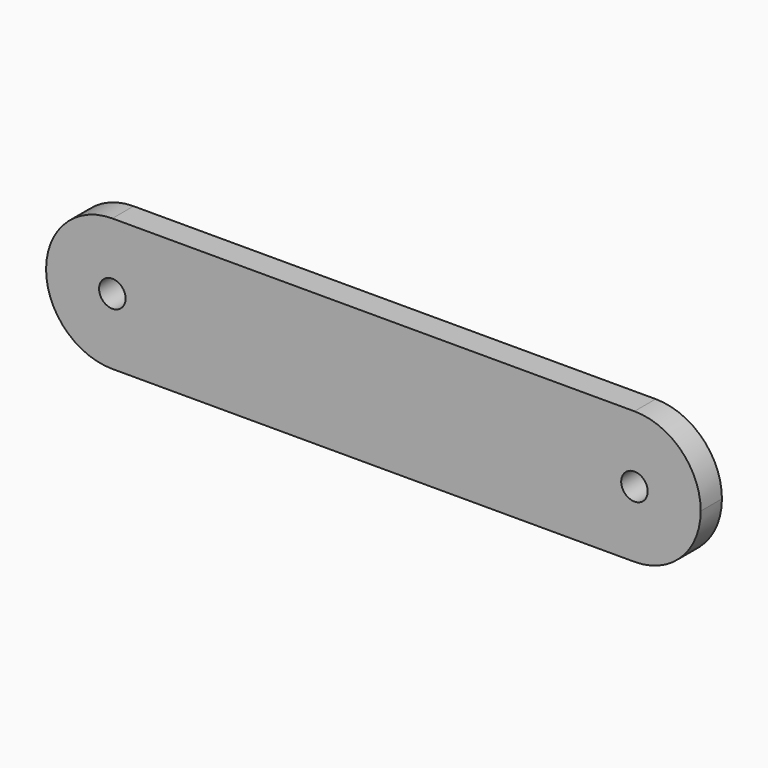
from build123d import *

# Parameters (mm, degrees)
F0_W     = 49.4
F0_H     = 10
F0_R     = 1
F1_DEPTH = 2
F2_R     = 4.99999


# Not quite as in the source:
# - a fillet or chamfer is up to 0.001 mm smaller than in the source, because OpenCascade refuses the exact size


with BuildPart() as f1:
    # F0 (on Front) → F1 (new body)
    with BuildSketch(Plane.XZ):
        with Locations((24.7, -5)):
            Rectangle(F0_W, F0_H)
        with Locations((5, -5)):
            Circle(F0_R, mode=Mode.SUBTRACT)
        with Locations((44.4, -5)):
            Circle(F0_R, mode=Mode.SUBTRACT)
    extrude(amount=F1_DEPTH)

    # F2 (radius 5 in the source; OpenCascade refuses exactly that, so slightly less here)
    f2_edges = [f1.edges().sort_by_distance(p)[0] for p in [
        (0, -1, 0),
        (0, -1, -10),
        (49.4, -1, 0),
        (49.4, -1, -10),
    ]]
    fillet(f2_edges, radius=F2_R)


solid = f1.part
